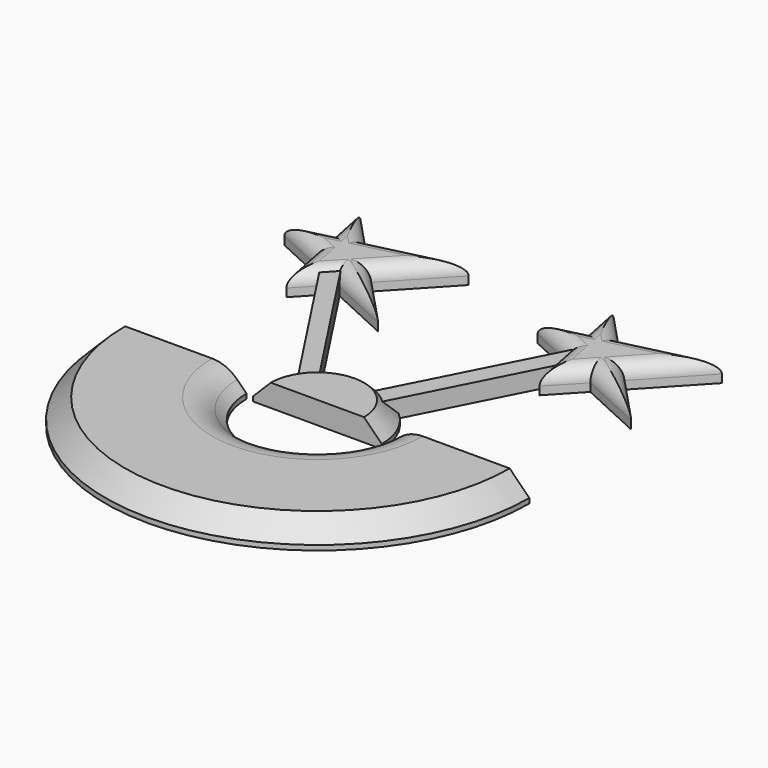
from build123d import *

# Parameters (mm, degrees)
F1_DEPTH  = 3.175
F3_SIZE   = 2.54
F3_2_SIZE = 2.54
F4_R      = 2.032
F4_2_R    = 2.032
F5_DEPTH  = 2.54
F6_SCALE  = 1.1
F7_R      = 5.08


with BuildPart() as f1:
    # F0 (on Top) → F1 (new body)
    with BuildSketch(Plane.XY):
        with BuildLine():
            Line((-9.1614854195, 0), (-27.3918092078, 0))
            ThreePointArc((-27.3918092078, 0), (0, -27.3918092078), (27.3918092078, 0))
            Line((27.3918092078, 0), (9.1614854195, 0))
            ThreePointArc((9.1614854195, 0), (0, -9.1614854195), (-9.1614854195, 0))
        make_face()
    extrude(amount=F1_DEPTH)

    # F3
    f3_edges = [f1.edges().sort_by_distance(p)[0] for p in [
        (0, -27.391809, 3.175),
        (0, -9.161485, 3.175),
    ]]
    chamfer(f3_edges, length=F3_SIZE)


with BuildPart() as f1b:
    # F0 (on Top) → F1, piece 2 (new body)
    with BuildSketch(Plane.XY):
        with BuildLine():
            ThreePointArc((9.1614854195, 0), (0, 9.1614854195), (-9.1614854195, 0))
            Line((-9.1614854195, 0), (9.1614854195, 0))
        make_face()
    extrude(amount=F1_DEPTH)

    # F3#2
    f3_2_edges = [f1b.edges().sort_by_distance(p)[0] for p in [
        (0, 9.161485, 3.175),
    ]]
    chamfer(f3_2_edges, length=F3_2_SIZE)



with BuildPart() as f1c:
    # F0 (on Top) → F1, piece 3 (new body)
    with BuildSketch(Plane.XY):
        Polygon((-24.1434442522, 32.9058568742), (-29.9002138344, 31.5146891815), (-23.2430197609, 28.446612912), (-21.9181837643, 21.8855220314), (-18.027946452, 26.043161475), (-8.8159006837, 21.7976402083), (-15.4235407651, 28.8265854518), (-7.9435985535, 36.8206743151), (-20.1626382848, 33.8678492857), (-25.4798094968, 39.5240449681), align=None)
    extrude(amount=F1_DEPTH)

    # F4
    f4_edges = [f1c.edges().sort_by_distance(p)[0] for p in [
        (-24.811627, 36.214951, 3.175),
        (-27.021829, 32.210273, 3.175),
        (-26.571617, 29.980651, 3.175),
        (-22.580602, 25.166067, 3.175),
        (-19.973065, 23.964342, 3.175),
        (-13.421924, 23.920401, 3.175),
        (-12.119721, 25.312113, 3.175),
        (-11.68357, 32.82363, 3.175),
        (-14.053118, 35.344262, 3.175),
        (-22.821224, 36.695947, 3.175),
    ]]
    fillet(f4_edges, radius=F4_R)


with BuildPart() as f1d:
    # F0 (on Top) → F1, piece 4 (new body)
    with BuildSketch(Plane.XY):
        Polygon((11.2036633424, 38.6662524052), (12.5400285869, 32.0480643113), (6.7832590048, 30.6568966185), (13.4404530783, 27.5888203491), (14.7652890749, 21.0277294685), (18.6555263872, 25.185368912), (27.8675721555, 20.9398476454), (21.2599320741, 27.9687928889), (28.7398742856, 35.9628817521), (16.5208345543, 33.0100567228), align=None)
    extrude(amount=F1_DEPTH)

    # F4#2
    f4_2_edges = [f1d.edges().sort_by_distance(p)[0] for p in [
        (11.871846, 35.357158, 3.175),
        (9.661644, 31.35248, 3.175),
        (10.111856, 29.122858, 3.175),
        (14.102871, 24.308275, 3.175),
        (16.710408, 23.106549, 3.175),
        (23.261549, 23.062608, 3.175),
        (24.563752, 24.45432, 3.175),
        (24.999903, 31.965837, 3.175),
        (22.630354, 34.486469, 3.175),
        (13.862249, 35.838155, 3.175),
    ]]
    fillet(f4_2_edges, radius=F4_2_R)


with BuildPart() as f1b_1:
    add(f1b.part)

    add(f1c.part)  # F5 merges F1c

    add(f1d.part)  # F5 merges F1d
    # F2 (on Top) → F5 (join)
    with BuildSketch(Plane.XY):
        Polygon((-2.0645700861, 2.2726482712), (-19.2176494747, 28.4420885146), (-21.1324576001, 27.1343351182), (-4.0035260891, 1.0017358657), align=None)
        Polygon((14.6486843005, 29.761556536), (1.0141873499, 3.0423374847), (3.3450562177, 1.6556362603), (17.0594274782, 28.5313832123), align=None)
    extrude(amount=F5_DEPTH)


with BuildPart() as f1_1:
    # F6: moved
    add(f1.part.scale(F6_SCALE))

    # F7
    f7_edges = [f1_1.edges().sort_by_distance(p)[0] for p in [
        (0, -12.871634, 3.4925),
    ]]
    fillet(f7_edges, radius=F7_R)


solid = Compound([f1b_1.part, f1_1.part])
